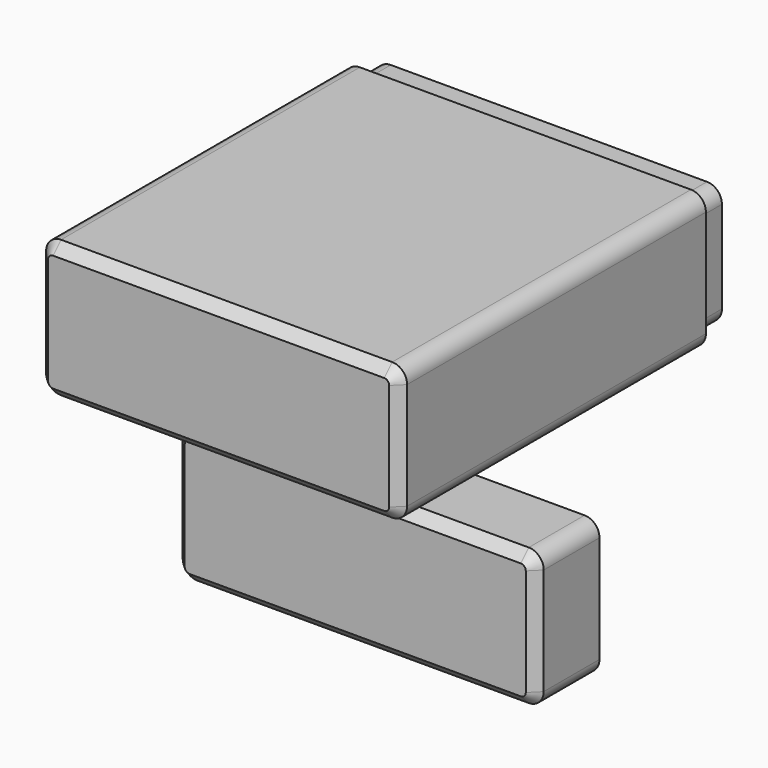
from build123d import *

# Parameters (mm, degrees)
F0_W       = 69.5
F0_H       = 89.25
F1_DEPTH   = 24.5
F2_W       = 67
F2_H       = 18
F3_DEPTH   = 87
F4_W       = 67
F4_H       = 3
F5_DEPTH   = 87
F6_W       = 72.5
F6_H       = 27.5
F6_W_2     = 69.5
F6_H_2     = 24.5
F7_DEPTH   = 77
F8_W       = 6.35
F8_H       = 24.5
F1_FACE3_W = 12.25
F1_FACE3_H = 24.5
F9_DEPTH   = 70
F10_W      = 72.5
F10_H      = 27.5
F11_DEPTH  = 16
F12_W      = 70
F12_H      = 25
F13_DEPTH  = 14
F14_R      = 3
F15_SIZE   = 2
F16_R      = 3
F17_SIZE   = 2
F18_R      = 3
F19_R      = 3


# Not quite as in the source:
# - a feature names something its author has since deleted; it is built from what else it names


with BuildPart() as f1:
    # F0 (on Top) → F1 (new body)
    with BuildSketch(Plane.XY):
        with Locations((-6.8625951707, 2.9138845081)):
            Rectangle(F0_W, F0_H)
    extrude(amount=F1_DEPTH)

    # F2 (on face) → F3 (cut)
    with BuildSketch(Plane(origin=(0, 47.5388845081, 0), x_dir=(-1, 0, 0), z_dir=(0, 1, 0))):
        with Locations((6.8625951707, 10.25)):
            Rectangle(F2_W, F2_H)
    extrude(amount=-F3_DEPTH, mode=Mode.SUBTRACT)

    # F4 (on face) → F5 (cut)
    with BuildSketch(Plane(origin=(0, 47.5388845081, 0), x_dir=(-1, 0, 0), z_dir=(0, 1, 0))):
        with Locations((6.8625951707, 21.75)):
            Rectangle(F4_W, F4_H)
    extrude(amount=-F5_DEPTH, mode=Mode.SUBTRACT)

    # F6 (on face) → F7 (join)
    with BuildSketch(Plane.XZ.offset(41.7111154919)):
        with Locations((-6.8625951707, 12.25)):
            Rectangle(F6_W, F6_H)
        with Locations((-6.8625951707, 12.25)):
            Rectangle(F6_W_2, F6_H_2, mode=Mode.SUBTRACT)
    extrude(amount=-F7_DEPTH)

    # F8 (on face) + F1_face3 (on face) → F9 (cut)
    with BuildSketch(Plane.YZ.offset(27.8874048293)):
        with Locations((44.3638845081, 12.25)):
            Rectangle(F8_W, F8_H)
    with BuildSketch(Plane(origin=(-41.6125951707, 41.4138845081, 12.25), x_dir=(0, -1, 0), z_dir=(-1, 0, 0))):
        Rectangle(F1_FACE3_W, F1_FACE3_H)
    extrude(amount=-F9_DEPTH, dir=(1, 0, 0), mode=Mode.SUBTRACT)

    # F16
    f16_edges = [f1.edges().sort_by_distance(p)[0] for p in [
        (29.387405, -3.211115, -1.5),
        (29.387405, -3.211115, 26),
        (-43.112595, -3.211115, -1.5),
        (-43.112595, -3.211115, 26),
    ]]
    fillet(f16_edges, radius=F16_R)

    # F17
    f17_edges = [f1.edges().sort_by_distance(p)[0] for p in [
        (-6.862595, -41.711115, 26),
        (28.508725, -41.711115, 25.12132),
        (-42.233916, -41.711115, 25.12132),
        (29.387405, -41.711115, 12.25),
        (-43.112595, -41.711115, 12.25),
        (28.508725, -41.711115, -0.62132),
        (-42.233916, -41.711115, -0.62132),
        (-6.862595, -41.711115, -1.5),
    ]]
    chamfer(f17_edges, length=F17_SIZE)

    # F18
    f18_edges = [f1.edges().sort_by_distance(p)[0] for p in [
        (-41.612595, 38.238885, 24.5),
        (27.887405, 38.238885, 24.5),
        (-41.612595, 38.238885, 0),
        (27.887405, 38.238885, 0),
    ]]
    fillet(f18_edges, radius=F18_R)


with BuildPart() as f11:
    # F10 (on Front) → F11 (new body)
    with BuildSketch(Plane.XZ):
        with Locations((0, -28.75)):
            Rectangle(F10_W, F10_H)
    extrude(amount=F11_DEPTH)

    # F12 (on face) → F13 (cut)
    with BuildSketch(Plane(origin=(0, 0, 0), x_dir=(-1, 0, 0), z_dir=(0, 1, 0))):
        with Locations((0, -28.75)):
            Rectangle(F12_W, F12_H)
    extrude(amount=-F13_DEPTH, mode=Mode.SUBTRACT)

    # F14
    f14_edges = [f11.edges().sort_by_distance(p)[0] for p in [
        (36.25, -8, -42.5),
        (-36.25, -8, -42.5),
        (-36.25, -8, -15),
        (36.25, -8, -15),
    ]]
    fillet(f14_edges, radius=F14_R)

    # F15
    f15_edges = [f11.edges().sort_by_distance(p)[0] for p in [
        (0, -16, -42.5),
    ]]
    chamfer(f15_edges, length=F15_SIZE)

    # F19
    f19_edges = [f11.edges().sort_by_distance(p)[0] for p in [
        (-35, -7, -16.25),
        (35, -7, -16.25),
        (-35, -7, -41.25),
        (35, -7, -41.25),
    ]]
    fillet(f19_edges, radius=F19_R)


solid = Compound([f1.part, f11.part])
